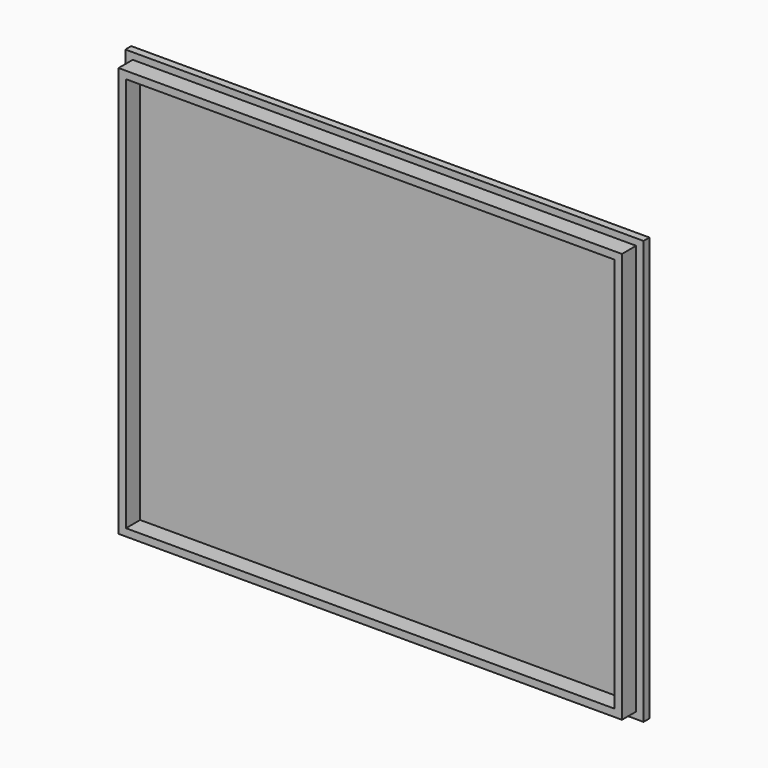
from build123d import *

# Parameters (mm, degrees)
F0_W        = 175
F0_H        = 143
F1_DEPTH    = 2.5
F2_W        = 170
F2_H        = 138.5
F3_DEPTH    = 6
F4_T        = 2.5
F4_T3_DEPTH = 175
F4_T5_DEPTH = 143.5


# Not quite as in the source:
# - a shell that OpenCascade refuses in one call is made with other operations: the cavity is built on its own and cut out


with BuildPart() as f1:
    # F0 (on Front) → F1 (new body)
    with BuildSketch(Plane.XZ):
        Rectangle(F0_W, F0_H)
    extrude(amount=F1_DEPTH)

    # F2 (on face) → F3 (join)
    with BuildSketch(Plane.XZ.offset(2.5)):
        Rectangle(F2_W, F2_H)
    extrude(amount=F3_DEPTH)

    # F4: shell of thickness 2.5, made by hand


with BuildPart() as f4_core1:
    # F4_t2: copy of F1
    add(f1.part)

    # the walls: a layer under each face that stays
    f4_faces = [f4_core1.faces().sort_by_distance(p)[0] for p in [
        (0, -1.25, -71.5),
        (-87.5, -1.25, 0),
        (87.5, -1.25, 0),
        (0, 0, 0),
        (60.15625, -2.5, -69.7345679012),
        (0, -1.25, 71.5),
        (0, -5.5, -69.25),
        (85, -5.5, 0),
        (0, -5.5, 69.25),
        (-85, -5.5, 0),
    ]]
    thicken(f4_faces, amount=-F4_T, mode=Mode.SUBTRACT)

    # F4_s4 → F4_t3 (cut)
    with BuildSketch(Plane.YZ.offset(-87.5)):
        Polygon((-2.525, -69.275), (0, -69.25), (0, -66.75), (-2.5, -66.75), align=None)
        Polygon((-2.525, 69.275), (0, 69.25), (0, 66.75), (-2.5, 66.75), align=None)
    extrude(amount=F4_T3_DEPTH, mode=Mode.SUBTRACT)

    # F4_s6 → F4_t5 (cut)
    with BuildSketch(Plane.XY.offset(-71.75)):
        Polygon((85.025, -2.525), (85, 0), (82.5, 0), (82.5, -2.5), align=None)
        Polygon((-85.025, -2.525), (-85, 0), (-82.5, 0), (-82.5, -2.5), align=None)
    extrude(amount=F4_T5_DEPTH, mode=Mode.SUBTRACT)


with BuildPart() as f1_1:
    add(f1.part)

    # what is left inside the walls is the cavity
    f4_cavity = [f4_core1.part.solids().sort_by_distance(p)[0] for p in [
        (0, -2.525, -22.25),
    ]]
    add(f4_cavity, mode=Mode.SUBTRACT)


solid = f1_1.part
